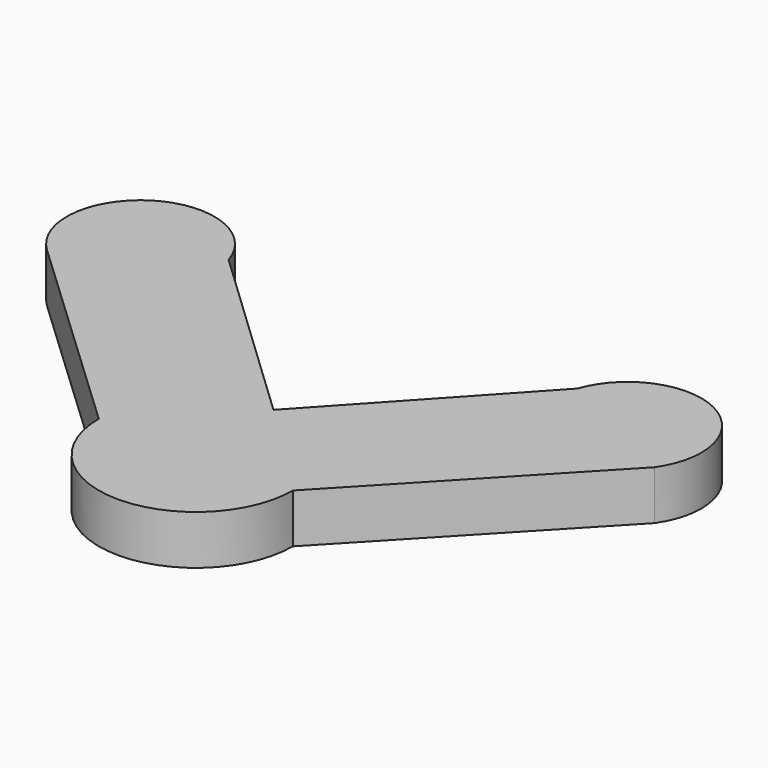
from build123d import *

# Parameters (mm, degrees)
F4_DEPTH = 5.08


# Not quite as in the source:
# - the program builds the solid bodies; features that only make, move or delete a surface that nothing else refers to are left out


with BuildPart() as f4:
    # F0 (on Top) → F4 (new body)
    with BuildSketch(Plane.XY):
        with BuildLine():
            ThreePointArc((0, 10.0203), (7.0854220795, 7.0854220795), (10.0203, 0))
            Line((10.0203, 0), (30.2514023598, 21.3797036526))
            ThreePointArc((30.2514023598, 21.3797036526), (27.4591098659, 32.5138598171), (16.8107412275, 28.2268356499))
            Line((16.8107412275, 28.2268356499), (0, 10.0203))
        make_face()
        with BuildLine():
            ThreePointArc((-10.0203, 0), (-7.0854220795, 7.0854220795), (0, 10.0203))
            Line((0, 10.0203), (-19.2001006115, 28.2268356499))
            ThreePointArc((-19.2001006115, 28.2268356499), (-30.5143757694, 32.4238900578), (-31.6996835172, 20.4145964235))
            Line((-31.6996835172, 20.4145964235), (-10.0203, 0))
        make_face()
        with BuildLine():
            ThreePointArc((-10.0203, 0), (0, -10.0203), (10.0203, 0))
            ThreePointArc((10.0203, 0), (7.0854220795, 7.0854220795), (0, 10.0203))
            ThreePointArc((0, 10.0203), (-7.0854220795, 7.0854220795), (-10.0203, 0))
        make_face()
    extrude(amount=F4_DEPTH)


solid = f4.part
